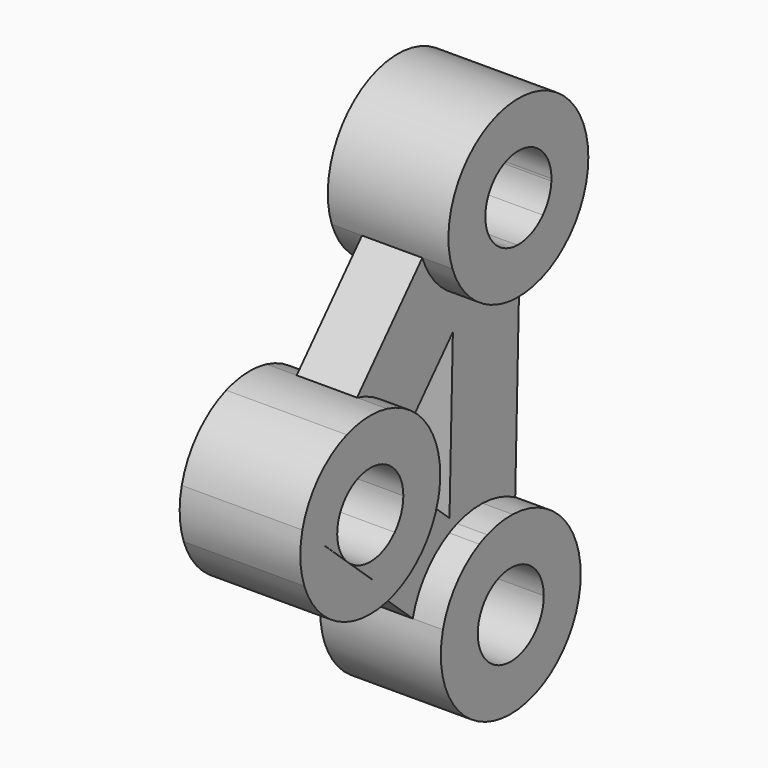
from build123d import *

# Parameters (mm, degrees)
F1_DEPTH = 10
F2_DEPTH = 5


with BuildPart() as f1:
    # F0 (on Right) → F1 (new body, symmetric)
    with BuildSketch(Plane.YZ):
        with BuildLine():
            Line((-0.468126, 9.67761), (3.510161, 14.060337))
            ThreePointArc((3.510161, 14.060337), (-0.700183, 14.474945), (-4.850853, 13.655897))
            Line((-4.850853, 13.655897), (-0.468126, 9.67761))
        make_face()
        with BuildLine():
            Line((-9.67761, -0.468126), (-14.060337, 3.510161))
            ThreePointArc((-14.060337, 3.510161), (-14.474945, -0.700183), (-13.655897, -4.850853))
            Line((-13.655897, -4.850853), (-9.67761, -0.468126))
        make_face()
        with BuildLine():
            ThreePointArc((-3.510161, -14.060337), (0.700183, -14.474945), (4.850853, -13.655897))
            Line((4.850853, -13.655897), (0.468126, -9.67761))
            Line((0.468126, -9.67761), (-3.510161, -14.060337))
        make_face()
        with BuildLine():
            ThreePointArc((4.850853, -13.655897), (4.865995, -13.650509), (4.88113, -13.645104))
            Line((4.88113, -13.645104), (0.487175, -9.656625))
            Line((0.487175, -9.656625), (0.468126, -9.67761))
            Line((0.468126, -9.67761), (4.850853, -13.655897))
        make_face()
        Polygon((-9.669191, -0.458852), (-14.060337, 3.510161), (-9.67761, -0.468126), align=None)
        with BuildLine():
            Line((-0.468126, 9.67761), (-4.850853, 13.655897))
            ThreePointArc((-4.850853, 13.655897), (-10.730436, 9.740228), (-14.060337, 3.510161))
            Line((-14.060337, 3.510161), (-9.669191, -0.458852))
            Line((-9.669191, -0.458852), (-5.072868, 4.604742))
            Line((-5.072868, 4.604742), (-0.468126, 9.67761))
        make_face()
        with BuildLine():
            ThreePointArc((-13.655897, -4.850853), (-9.740228, -10.730436), (-3.510161, -14.060337))
            Line((-3.510161, -14.060337), (0.468126, -9.67761))
            Line((0.468126, -9.67761), (-4.604742, -5.072868))
            Line((-4.604742, -5.072868), (-9.67761, -0.468126))
            Line((-9.67761, -0.468126), (-13.655897, -4.850853))
        make_face()
        with BuildLine():
            Line((9.67761, 0.468126), (13.655897, 4.850853))
            ThreePointArc((13.655897, 4.850853), (9.740228, 10.730436), (3.510161, 14.060337))
            Line((3.510161, 14.060337), (-0.468126, 9.67761))
            Line((-0.468126, 9.67761), (4.604742, 5.072868))
            Line((4.604742, 5.072868), (9.67761, 0.468126))
        make_face()
        with BuildLine():
            ThreePointArc((4.88113, -13.645104), (10.741232, -9.728322), (14.060337, -3.510161))
            Line((14.060337, -3.510161), (9.67761, 0.468126))
            Line((9.67761, 0.468126), (9.252682, 0))
            Line((9.252682, 0), (5.072868, -4.604742))
            Line((5.072868, -4.604742), (0.487175, -9.656625))
            Line((0.487175, -9.656625), (4.88113, -13.645104))
        make_face()
        with BuildLine():
            Line((9.252682, 0), (9.67761, 0.468126))
            Line((9.67761, 0.468126), (4.604742, 5.072868))
            ThreePointArc((4.604742, 5.072868), (6.264391, 2.773992), (6.851105, 0))
            ThreePointArc((6.851105, 0), (6.391103, -2.468085), (5.072868, -4.604742))
            Line((5.072868, -4.604742), (9.252682, 0))
        make_face()
        with BuildLine():
            Line((4.604742, 5.072868), (-0.468126, 9.67761))
            Line((-0.468126, 9.67761), (-5.072868, 4.604742))
            ThreePointArc((-5.072868, 4.604742), (-0.331015, 6.843103), (4.604742, 5.072868))
        make_face()
        with BuildLine():
            Line((-4.124752, -5.470288), (0.487175, -9.656625))
            Line((0.487175, -9.656625), (5.072868, -4.604742))
            ThreePointArc((5.072868, -4.604742), (0.641891, -6.820968), (-4.124752, -5.470288))
        make_face()
        with BuildLine():
            ThreePointArc((-5.026979, -4.654795), (-6.85102, -0.033953), (-5.072868, 4.604742))
            Line((-5.072868, 4.604742), (-9.669191, -0.458852))
            Line((-9.669191, -0.458852), (-5.026979, -4.654795))
        make_face()
        with BuildLine():
            ThreePointArc((14.060337, -3.510161), (14.383582, -1.768294), (14.49187, 0))
            ThreePointArc((14.49187, 0), (14.281348, 2.46118), (13.655897, 4.850853))
            Line((13.655897, 4.850853), (9.67761, 0.468126))
            Line((9.67761, 0.468126), (14.060337, -3.510161))
        make_face()
    extrude(amount=F1_DEPTH, both=True)


with BuildPart() as f1b:
    # F0 (on Right) → F1, piece 2 (new body, symmetric)
    with BuildSketch(Plane.YZ):
        with BuildLine():
            Line((24.518737, -31.470545), (15.057521, -22.882413))
            ThreePointArc((15.057521, -22.882413), (27.337683, -40.790769), (43.605825, -26.40817))
            ThreePointArc((43.605825, -26.40817), (41.642383, -19.124436), (36.284094, -13.814386))
            Line((36.284094, -13.814386), (35.950889, -26.40817))
            ThreePointArc((35.950889, -26.40817), (31.88221, -32.659604), (24.518737, -31.470545))
        make_face()
        with BuildLine():
            ThreePointArc((22.611773, -13.456879), (17.805801, -17.34506), (15.057521, -22.882413))
            Line((15.057521, -22.882413), (24.518737, -31.470545))
            ThreePointArc((24.518737, -31.470545), (22.827035, -29.094862), (22.279335, -26.230294))
            Line((22.279335, -26.230294), (22.611773, -13.456879))
        make_face()
        with BuildLine():
            Line((29.493839, -11.92128), (29.350453, -17.3893))
            Line((29.350453, -17.3893), (33.709172, -21.345794))
            ThreePointArc((33.709172, -21.345794), (35.365389, -23.639915), (35.950889, -26.40817))
            Line((35.950889, -26.40817), (36.284094, -13.814386))
            ThreePointArc((36.284094, -13.814386), (33.005828, -12.44867), (29.493839, -11.92128))
        make_face()
        with BuildLine():
            Line((29.350453, -17.3893), (24.247955, -12.757662))
            ThreePointArc((24.247955, -12.757662), (23.419123, -13.082136), (22.611773, -13.456879))
            Line((22.611773, -13.456879), (22.279335, -26.230294))
            ThreePointArc((22.279335, -26.230294), (24.407414, -21.449123), (29.293175, -19.573585))
            Line((29.293175, -19.573585), (29.350453, -17.3893))
        make_face()
        with BuildLine():
            ThreePointArc((29.493839, -11.92128), (26.832247, -12.097051), (24.247955, -12.757662))
            Line((24.247955, -12.757662), (29.350453, -17.3893))
            Line((29.350453, -17.3893), (29.493839, -11.92128))
        make_face()
        with BuildLine():
            Line((33.709172, -21.345794), (29.350453, -17.3893))
            Line((29.350453, -17.3893), (29.293175, -19.573585))
            ThreePointArc((29.293175, -19.573585), (31.660324, -20.063119), (33.709172, -21.345794))
        make_face()
    extrude(amount=F1_DEPTH, both=True)


with BuildPart() as f1c:
    # F0 (on Right) → F1, piece 3 (new body, symmetric)
    with BuildSketch(Plane.YZ):
        with BuildLine():
            ThreePointArc((45.184994, 33.813442), (28.231944, 48.094789), (17.037227, 28.962588))
            Line((17.037227, 28.962588), (25.620256, 38.418183))
            ThreePointArc((25.620256, 38.418183), (33.161209, 40.204544), (37.544229, 33.813442))
            ThreePointArc((37.544229, 33.813442), (37.541832, 33.632239), (37.534643, 33.451163))
            Line((37.534643, 33.451163), (37.201648, 20.865337))
            ThreePointArc((37.201648, 20.865337), (43.028743, 26.207733), (45.184994, 33.813442))
        make_face()
        with BuildLine():
            Line((25.620256, 38.418183), (17.037227, 28.962588))
            ThreePointArc((17.037227, 28.962588), (19.580527, 24.511587), (23.514384, 21.224558))
            Line((23.514384, 21.224558), (23.842019, 33.813442))
            ThreePointArc((23.842019, 33.813442), (24.302021, 36.281527), (25.620256, 38.418183))
        make_face()
        with BuildLine():
            ThreePointArc((23.514384, 21.224558), (25.29827, 20.363168), (27.182963, 19.753105))
            Line((27.182963, 19.753105), (30.417877, 23.316886))
            Line((30.417877, 23.316886), (30.513532, 26.964691))
            ThreePointArc((30.513532, 26.964691), (25.785577, 29.032896), (23.842019, 33.813442))
            Line((23.842019, 33.813442), (23.514384, 21.224558))
        make_face()
        with BuildLine():
            Line((35.765992, 29.2087), (30.417877, 23.316886))
            Line((30.417877, 23.316886), (30.31324, 19.326551))
            ThreePointArc((30.31324, 19.326551), (33.852558, 19.670165), (37.201648, 20.865337))
            Line((37.201648, 20.865337), (37.534643, 33.451163))
            ThreePointArc((37.534643, 33.451163), (37.016713, 31.177184), (35.765992, 29.2087))
        make_face()
        with BuildLine():
            Line((30.417877, 23.316886), (27.182963, 19.753105))
            ThreePointArc((27.182963, 19.753105), (28.736443, 19.454274), (30.31324, 19.326551))
            Line((30.31324, 19.326551), (30.417877, 23.316886))
        make_face()
        with BuildLine():
            Line((30.513532, 26.964691), (30.417877, 23.316886))
            Line((30.417877, 23.316886), (35.765992, 29.2087))
            ThreePointArc((35.765992, 29.2087), (33.384765, 27.513227), (30.513532, 26.964691))
        make_face()
    extrude(amount=F1_DEPTH, both=True)


with BuildPart() as f2:
    # F0 (on Right) → F2 (new body, symmetric)
    with BuildSketch(Plane.YZ):
        with BuildLine():
            ThreePointArc((37.201648, 20.865337), (33.852558, 19.670165), (30.31324, 19.326551))
            Line((30.31324, 19.326551), (29.493839, -11.92128))
            ThreePointArc((29.493839, -11.92128), (33.005828, -12.44867), (36.284094, -13.814386))
            Line((36.284094, -13.814386), (37.201648, 20.865337))
        make_face()
        with BuildLine():
            Line((27.182963, 19.753105), (23.366669, 15.54884))
            Line((23.366669, 15.54884), (22.667312, -11.322881))
            Line((22.667312, -11.322881), (24.247955, -12.757662))
            ThreePointArc((24.247955, -12.757662), (26.832247, -12.097051), (29.493839, -11.92128))
            Line((29.493839, -11.92128), (30.31324, 19.326551))
            ThreePointArc((30.31324, 19.326551), (28.736443, 19.454274), (27.182963, 19.753105))
        make_face()
        with BuildLine():
            Line((22.667312, -11.322881), (14.060337, -3.510161))
            ThreePointArc((14.060337, -3.510161), (10.741232, -9.728322), (4.88113, -13.645104))
            Line((4.88113, -13.645104), (15.057521, -22.882413))
            ThreePointArc((15.057521, -22.882413), (17.805801, -17.34506), (22.611773, -13.456879))
            Line((22.611773, -13.456879), (22.667312, -11.322881))
        make_face()
        with BuildLine():
            ThreePointArc((3.510161, 14.060337), (9.740228, 10.730436), (13.655897, 4.850853))
            Line((13.655897, 4.850853), (23.366669, 15.54884))
            Line((23.366669, 15.54884), (23.514384, 21.224558))
            ThreePointArc((23.514384, 21.224558), (19.580527, 24.511587), (17.037227, 28.962588))
            Line((17.037227, 28.962588), (3.510161, 14.060337))
        make_face()
        with BuildLine():
            Line((23.514384, 21.224558), (23.366669, 15.54884))
            Line((23.366669, 15.54884), (27.182963, 19.753105))
            ThreePointArc((27.182963, 19.753105), (25.29827, 20.363168), (23.514384, 21.224558))
        make_face()
        with BuildLine():
            Line((24.247955, -12.757662), (22.667312, -11.322881))
            Line((22.667312, -11.322881), (22.611773, -13.456879))
            ThreePointArc((22.611773, -13.456879), (23.419123, -13.082136), (24.247955, -12.757662))
        make_face()
    extrude(amount=F2_DEPTH, both=True)


solid = Compound([f1.part, f1b.part, f1c.part, f2.part])
